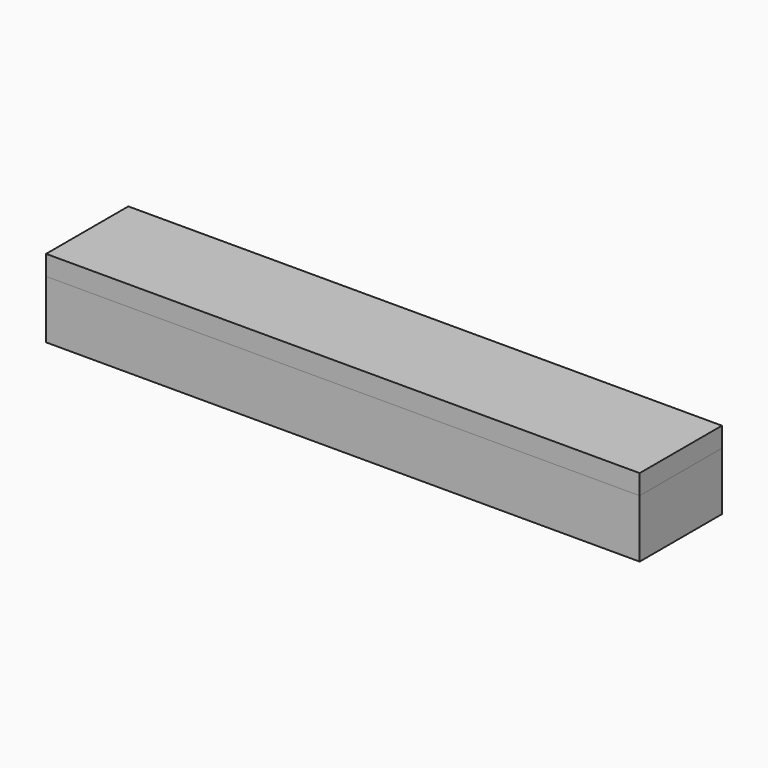
from build123d import *

# Parameters (mm, degrees)
F0_W     = 1136.65
F0_H     = 196.85
F0_W_2   = 1117.6
F0_H_2   = 177.8
F1_DEPTH = 111.125
F2_DEPTH = 38.1
F3_T     = -9.525
F3_2_T   = -9.525


# Not quite as in the source:
# - a feature of the source that left no trace in its solid (it failed there, or was rolled back) is left out


with BuildPart() as f1:
    # F0 (on Top) → F1 (new body)
    with BuildSketch(Plane.XY):
        Rectangle(F0_W, F0_H)
        Rectangle(F0_W_2, F0_H_2, mode=Mode.SUBTRACT)
        Rectangle(F0_W_2, F0_H_2)
    extrude(amount=F1_DEPTH)


with BuildPart() as f2:
    # F2 (new): a face of the model
    f2_faces = [f1.part.faces().sort_by_distance(p)[0] for p in [
        (0, 0, 111.125),
    ]]
    extrude(f2_faces, amount=F2_DEPTH)

    # F3#2
    f3_2_openings = [f2.faces().sort_by_distance(p)[0] for p in [
        (0, 0, 111.125),
    ]]
    offset(amount=F3_2_T, openings=f3_2_openings)


with BuildPart() as f1_1:
    add(f1.part)

    # F3
    f3_openings = [f1_1.faces().sort_by_distance(p)[0] for p in [
        (0, 0, 111.125),
    ]]
    offset(amount=F3_T, openings=f3_openings)


solid = Compound([f2.part, f1_1.part])
